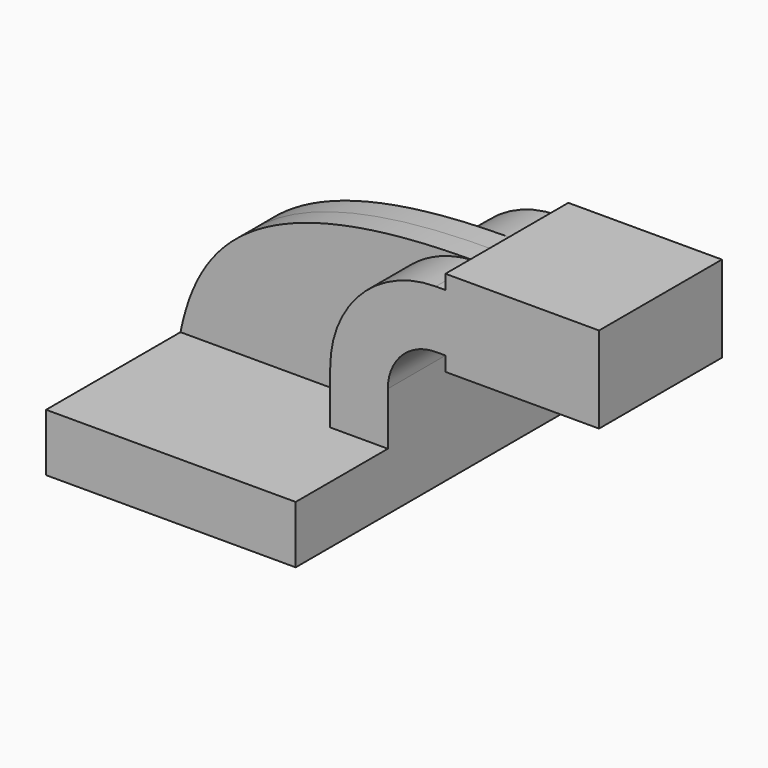
from build123d import *

# Parameters (mm, degrees)
F1_DEPTH = 63.5
F0_W     = 25.4
F0_H     = 28.575
F2_DEPTH = 25.4
F3_DEPTH = 7.9375


# Not quite as in the source:
# - a feature of the source that left no trace in its solid (it failed there, or was rolled back) is left out


with BuildPart() as f1:
    # F0 (on Front) → F1 (new body, symmetric)
    with BuildSketch(Plane.XZ):
        Polygon((-41.275, -9.525), (41.275, -9.525), (41.275, 9.525), (22.225, 9.525), (-41.275, 9.525), align=None)
    extrude(amount=F1_DEPTH, both=True)

    # F0 (on Front) → F2 (join, symmetric)
    with BuildSketch(Plane.XZ):
        Polygon((60.325, 66.675), (60.325, 61.9252), (60.325, 42.8752), (60.325, 38.1), (85.725, 38.1), (85.725, 66.675), align=None)
        with BuildLine():
            Line((22.225, 9.525), (41.275, 9.525))
            Line((41.275, 9.525), (41.275, 27.0002))
            ThreePointArc((41.275, 27.0002), (45.9246798487, 38.2255201513), (57.15, 42.8752))
            Line((57.15, 42.8752), (60.325, 42.8752))
            Line((60.325, 42.8752), (60.325, 61.9252))
            Line((60.325, 61.9252), (57.15, 61.9252))
            ThreePointArc((57.15, 61.9252), (32.4542956671, 51.6959043329), (22.225, 27.0002))
            Line((22.225, 27.0002), (22.225, 9.525))
        make_face()
        with Locations((98.425, 52.3875)):
            Rectangle(F0_W, F0_H)
    extrude(amount=F2_DEPTH, both=True)

    # F0 (on Front) → F3 (join, symmetric)
    with BuildSketch(Plane.XZ):
        with BuildLine():
            add(Edge.make_bspline(
                [(60.325, 61.9252), (-18.8444089144, 62.9406571388), (-35.6957179924, 36.5767096935), (-41.275, 9.525)],
                knots=[0, 0, 0, 0, 114.3168446032, 114.3168446032, 114.3168446032, 114.3168446032], degree=3))
            Line((-41.275, 9.525), (22.225, 9.525))
            Line((22.225, 9.525), (22.225, 27.0002))
            ThreePointArc((22.225, 27.0002), (32.4542956671, 51.6959043329), (57.15, 61.9252))
            Line((57.15, 61.9252), (60.325, 61.9252))
        make_face()
    extrude(amount=F3_DEPTH, both=True)


solid = f1.part
